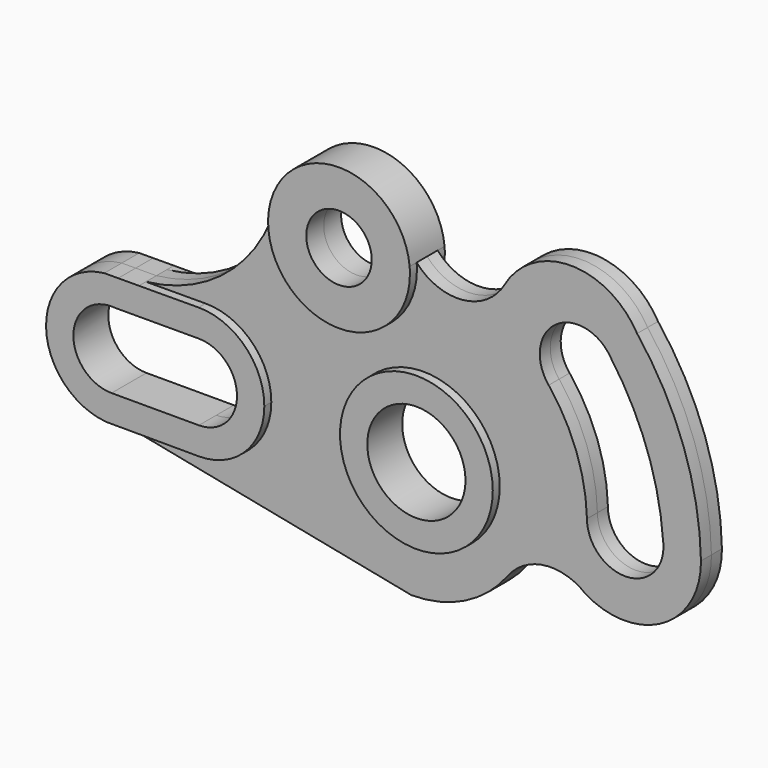
from build123d import *

# Parameters (mm, degrees)
F0_R     = 22.225
F1_DEPTH = 3.81
F2_DEPTH = 6.35
F0_R_2   = 9.525
F0_R_3   = 14.2875


with BuildPart() as f1:
    # F0 (on Front) → F1 (new body, symmetric)
    with BuildSketch(Plane.XZ):
        with BuildLine():
            Line((-71.2302067148, -19.0499547752), (-95.1790091363, -18.9977704048))
            ThreePointArc((-95.1790091363, -18.9977704048), (-96.6302067148, -19.0499547752), (-98.0811630947, -18.9914466199))
            Line((-98.0811630947, -18.9914466199), (-11.3598450249, -36.1872298845))
            ThreePointArc((-11.3598450249, -36.1872298845), (4.2709346458, -32.4941742986), (16.5960399757, -22.1960331421))
            ThreePointArc((16.5960399757, -22.1960331421), (27.4429735853, -15.9457724279), (39.4467694666, -19.4997296822))
            ThreePointArc((39.4467694666, -19.4997296822), (61.8517288175, -19.5048009495), (72.8764723136, 0))
            ThreePointArc((72.8764723136, 0), (67.8374893071, 27.6050269049), (54.2986201889, 52.1840399681))
            ThreePointArc((54.2986201889, 52.1840399681), (35.0247812601, 63.3424344385), (15.7509423313, 52.1840399681))
            ThreePointArc((15.7509423313, 52.1840399681), (3.628009846, 44.2991231357), (-9.8592897487, 49.517375251))
            ThreePointArc((-9.8592897487, 49.517375251), (-9.7940926646, 48.5721857626), (-9.7723450249, 47.625))
            ThreePointArc((-9.7723450249, 47.625), (-31.9572082975, 27.0455910398), (-50.8153078986, 50.7110154181))
            ThreePointArc((-50.8153078986, 50.7110154181), (-64.9081681748, 29.1142899479), (-88.6201192568, 18.9767045507))
            Line((-88.6201192568, 18.9767045507), (-71.2689823238, 19.0498308196))
            ThreePointArc((-71.2689823238, 19.0498308196), (-57.7467278848, 13.4987395145), (-52.1386969191, 0))
            ThreePointArc((-52.1386969191, 0), (-57.7329966699, -13.4850521246), (-71.2302067148, -19.0499547752))
        make_face()
        with Locations((-7.8918969191, 0)):
            Circle(F0_R, mode=Mode.SUBTRACT)
        with BuildLine():
            ThreePointArc((61.9581030809, 0), (50.8329030809, -11.1252), (39.7077030809, 0))
            ThreePointArc((39.7077030809, 0), (36.6426092928, 16.2092346589), (28.5715121556, 30.596433106))
            ThreePointArc((28.5715121556, 30.596433106), (29.9427690789, 46.2699714599), (45.6163074327, 44.8987145366))
            ThreePointArc((45.6163074327, 44.8987145366), (46.0483474014, 44.3497039456), (46.4450767121, 43.7746587147))
            ThreePointArc((46.4450767121, 43.7746587147), (57.1198457607, 23.6623392132), (61.8704480271, 1.3937993402))
            ThreePointArc((61.8704480271, 1.3937993402), (61.9361676926, 0.6982764512), (61.9581030809, 0))
        make_face(mode=Mode.SUBTRACT)
    extrude(amount=F1_DEPTH, both=True)


with BuildPart() as f2:
    # F0 (on Front) → F2 (new body, symmetric)
    with BuildSketch(Plane.XZ):
        with BuildLine():
            ThreePointArc((-96.5886969191, -11.0998), (-107.6764020371, -0.5180301702), (-97.6236283177, 11.0514468302))
            ThreePointArc((-97.6236283177, 11.0514468302), (-96.6090077674, 11.0997814172), (-95.5942171229, 11.0551603324))
            Line((-95.5942171229, 11.0551603324), (-86.6911309222, 11.0714515751))
            ThreePointArc((-86.6911309222, 11.0714515751), (-85.3763591725, 12.7126999407), (-83.8886969191, 14.1990316571))
            ThreePointArc((-83.8886969191, 14.1990316571), (-88.8942032902, 17.4269121704), (-94.6518588651, 18.9512838181))
            Line((-94.6518588651, 18.9512838181), (-98.6852034909, 18.9342853098))
            ThreePointArc((-98.6852034909, 18.9342853098), (-115.6362812002, -0.3033695006), (-98.0811630947, -18.9914466199))
            Line((-98.0811630947, -18.9914466199), (-95.1790091363, -18.9977704048))
            ThreePointArc((-95.1790091363, -18.9977704048), (-89.1369994129, -17.5321049585), (-83.8886969191, -14.1990316571))
            ThreePointArc((-83.8886969191, -14.1990316571), (-85.3647221317, -12.7256751951), (-86.6708459935, -11.0998))
            Line((-86.6708459935, -11.0998), (-96.5886969191, -11.0998))
        make_face()
        with BuildLine():
            Line((-81.1065478448, -11.0998), (-86.6708459935, -11.0998))
            ThreePointArc((-86.6708459935, -11.0998), (-85.3647221317, -12.7256751951), (-83.8886969191, -14.1990316571))
            ThreePointArc((-83.8886969191, -14.1990316571), (-82.4126717065, -12.7256751951), (-81.1065478448, -11.0998))
        make_face()
        with BuildLine():
            ThreePointArc((-83.8886969191, 14.1990316571), (-85.3763591725, 12.7126999407), (-86.6911309222, 11.0714515751))
            Line((-86.6911309222, 11.0714515751), (-81.0935830583, 11.0816942043))
            ThreePointArc((-81.0935830583, 11.0816942043), (-82.4052361424, 12.7173873258), (-83.8886969191, 14.1990316571))
        make_face()
        with BuildLine():
            Line((-71.1886969191, -11.0998), (-81.1065478448, -11.0998))
            ThreePointArc((-81.1065478448, -11.0998), (-82.4126717065, -12.7256751951), (-83.8886969191, -14.1990316571))
            ThreePointArc((-83.8886969191, -14.1990316571), (-78.0055423584, -17.7885670659), (-71.2302067148, -19.0499547752))
            ThreePointArc((-71.2302067148, -19.0499547752), (-57.7329966699, -13.4850521246), (-52.1386969191, 0))
            ThreePointArc((-52.1386969191, 0), (-57.7467278848, 13.4987395145), (-71.2689823238, 19.0498308196))
            ThreePointArc((-71.2689823238, 19.0498308196), (-78.0236429237, 17.7816200925), (-83.8886969191, 14.1990316571))
            ThreePointArc((-83.8886969191, 14.1990316571), (-82.4052361424, 12.7173873258), (-81.0935830583, 11.0816942043))
            Line((-81.0935830583, 11.0816942043), (-71.2090077674, 11.0997814172))
            ThreePointArc((-71.2090077674, 11.0997814172), (-63.3471373266, 7.8559215371), (-60.0888969191, 0))
            ThreePointArc((-60.0888969191, 0), (-63.3399530693, -7.8487438498), (-71.1886969191, -11.0998))
        make_face()
        with BuildLine():
            ThreePointArc((-71.2302067148, -19.0499547752), (-78.0055423584, -17.7885670659), (-83.8886969191, -14.1990316571))
            ThreePointArc((-83.8886969191, -14.1990316571), (-89.1369994129, -17.5321049585), (-95.1790091363, -18.9977704048))
            Line((-95.1790091363, -18.9977704048), (-71.2302067148, -19.0499547752))
        make_face()
        with BuildLine():
            ThreePointArc((-94.6518588651, 18.9512838181), (-88.8942032902, 17.4269121704), (-83.8886969191, 14.1990316571))
            ThreePointArc((-83.8886969191, 14.1990316571), (-78.0236429237, 17.7816200925), (-71.2689823238, 19.0498308196))
            Line((-71.2689823238, 19.0498308196), (-88.6201192568, 18.9767045507))
            Line((-88.6201192568, 18.9767045507), (-94.6518588651, 18.9512838181))
        make_face()
    extrude(amount=F2_DEPTH, both=True)


with BuildPart() as f2b:
    # F0 (on Front) → F2, piece 2 (new body, symmetric)
    with BuildSketch(Plane.XZ):
        with BuildLine():
            ThreePointArc((-9.8592897487, 49.517375251), (-29.8086319483, 68.2537408507), (-50.8153078986, 50.7110154181))
            ThreePointArc((-50.8153078986, 50.7110154181), (-31.9572082975, 27.0455910398), (-9.7723450249, 47.625))
            ThreePointArc((-9.7723450249, 47.625), (-9.7940926646, 48.5721857626), (-9.8592897487, 49.517375251))
        make_face()
        with Locations((-30.4098450249, 47.625)):
            Circle(F0_R_2, mode=Mode.SUBTRACT)
    extrude(amount=F2_DEPTH, both=True)


with BuildPart() as f2c:
    # F0 (on Front) → F2, piece 3 (new body, symmetric)
    with BuildSketch(Plane.XZ):
        with Locations((-7.8918969191, 0)):
            Circle(F0_R)
        with Locations((-7.8918969191, 0)):
            Circle(F0_R_3, mode=Mode.SUBTRACT)
    extrude(amount=F2_DEPTH, both=True)


solid = Compound([f1.part, f2.part, f2b.part, f2c.part])
